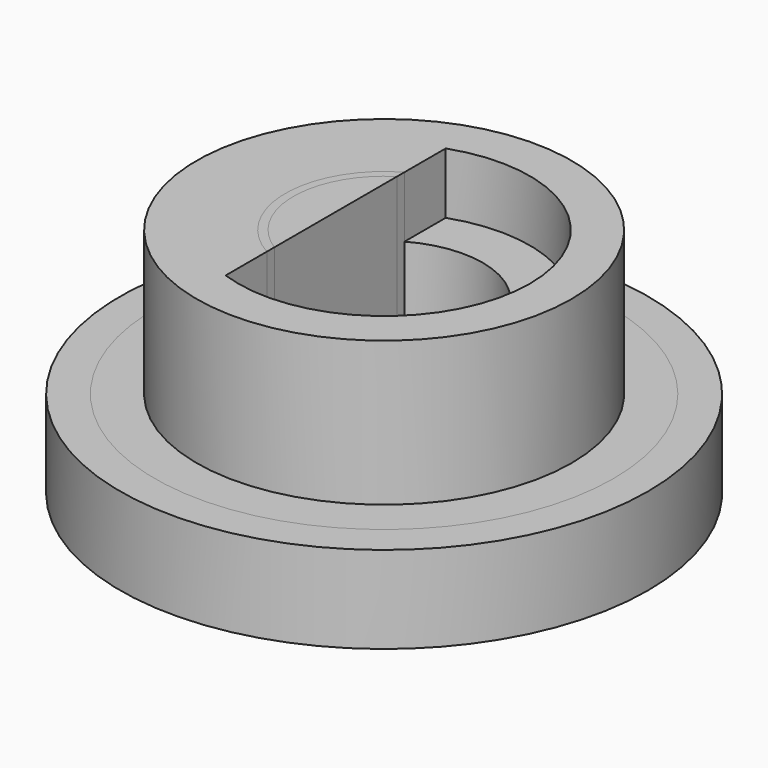
from build123d import *
from build123d import SkipClean  # not in build123d's __all__

# Parameters (mm, degrees)
F1_DEPTH      = 3
F1_DEPTH_BACK = 1
F0_R          = 6.75
F2_DEPTH      = 5.2
F2_DEPTH_BACK = 1
F0_R_2        = 8.26
F3_DEPTH      = 1
F0_R_3        = 9.505
F4_DEPTH      = 3.14
F5_DEPTH      = 5.2
F6_DEPTH      = 5.2
F6_DEPTH_BACK = 1


with BuildPart() as f1:
    # F0 (on Top) → F1 (new body, two sides)
    with BuildSketch(Plane.XY) as f1_sk:
        with BuildLine():
            ThreePointArc((-1.745, 3.0972568508), (1.7936763922, 3.0693240298), (3.555, 0))
            ThreePointArc((3.555, 0), (1.7936763922, -3.0693240298), (-1.745, -3.0972568508))
            Line((-1.745, -3.0972568508), (-1.745, -4.9515123952))
            ThreePointArc((-1.745, -4.9515123952), (3.0332532041, -4.2850758453), (5.25, 0))
            ThreePointArc((5.25, 0), (3.0332532041, 4.2850758453), (-1.745, 4.9515123952))
            Line((-1.745, 4.9515123952), (-1.745, 3.0972568508))
        make_face()
    extrude(amount=F1_DEPTH)
    extrude(f1_sk.sketch, amount=-F1_DEPTH_BACK)

    # F0 (on Top) → F2 (join, two sides)
    with BuildSketch(Plane.XY) as f2_sk:
        Circle(F0_R)
        with BuildLine():
            ThreePointArc((-1.745, -4.9515123952), (-5.25, 0), (-1.745, 4.9515123952))
            ThreePointArc((-1.745, 4.9515123952), (3.0332532041, 4.2850758453), (5.25, 0))
            ThreePointArc((5.25, 0), (3.0332532041, -4.2850758453), (-1.745, -4.9515123952))
        make_face(mode=Mode.SUBTRACT)
        with BuildLine():
            ThreePointArc((-1.745, -3.0972568508), (-3.555, 0), (-1.745, 3.0972568508))
            Line((-1.745, 3.0972568508), (-1.745, 4.9515123952))
            ThreePointArc((-1.745, 4.9515123952), (-5.25, 0), (-1.745, -4.9515123952))
            Line((-1.745, -4.9515123952), (-1.745, -3.0972568508))
        make_face()
    with SkipClean():  # cleaning this boolean's faces spoils the solid; the shape is the same uncleaned
        extrude(amount=F2_DEPTH)
        extrude(f2_sk.sketch, amount=-F2_DEPTH_BACK)


with BuildPart() as f3:
    # F0 (on Top) → F3 (new body)
    with BuildSketch(Plane.XY):
        Circle(F0_R_2)
        Circle(F0_R, mode=Mode.SUBTRACT)
    extrude(amount=-F3_DEPTH)


with BuildPart() as f3b:
    # F0 (on Top) → F3, piece 2 (new body)
    with BuildSketch(Plane.XY):
        with BuildLine():
            Line((-1.745, 0), (2.48, 0))
            ThreePointArc((2.48, 0), (0.9546727188, 2.288886192), (-1.745, 1.7622074225))
            Line((-1.745, 1.7622074225), (-1.745, 0))
        make_face()
        with BuildLine():
            Line((3.265, 0), (3.555, 0))
            ThreePointArc((3.555, 0), (1.7936763922, 3.0693240298), (-1.745, 3.0972568508))
            Line((-1.745, 3.0972568508), (-1.745, 2.7595651831))
            ThreePointArc((-1.745, 2.7595651831), (1.5752460125, 2.8598645073), (3.265, 0))
        make_face()
        with BuildLine():
            ThreePointArc((-1.745, -1.7622074225), (0.9546727188, -2.288886192), (2.48, 0))
            Line((2.48, 0), (-1.745, 0))
            Line((-1.745, 0), (-1.745, -1.7622074225))
        make_face()
        with BuildLine():
            ThreePointArc((-1.745, -2.7595651831), (1.5752460125, -2.8598645073), (3.265, 0))
            Line((3.265, 0), (2.48, 0))
            ThreePointArc((2.48, 0), (0.9546727188, -2.288886192), (-1.745, -1.7622074225))
            Line((-1.745, -1.7622074225), (-1.745, -2.7595651831))
        make_face()
        with BuildLine():
            Line((-1.745, 0), (-1.745, 1.7622074225))
            ThreePointArc((-1.745, 1.7622074225), (-2.48, 0), (-1.745, -1.7622074225))
            Line((-1.745, -1.7622074225), (-1.745, 0))
        make_face()
        with BuildLine():
            Line((-1.745, 1.7622074225), (-1.745, 2.7595651831))
            ThreePointArc((-1.745, 2.7595651831), (-3.265, 0), (-1.745, -2.7595651831))
            Line((-1.745, -2.7595651831), (-1.745, -1.7622074225))
            ThreePointArc((-1.745, -1.7622074225), (-2.48, 0), (-1.745, 1.7622074225))
        make_face()
        with BuildLine():
            ThreePointArc((-1.745, -3.0972568508), (1.7936763922, -3.0693240298), (3.555, 0))
            Line((3.555, 0), (3.265, 0))
            ThreePointArc((3.265, 0), (1.5752460125, -2.8598645073), (-1.745, -2.7595651831))
            Line((-1.745, -2.7595651831), (-1.745, -3.0972568508))
        make_face()
        with BuildLine():
            Line((2.48, 0), (3.265, 0))
            ThreePointArc((3.265, 0), (1.5752460125, 2.8598645073), (-1.745, 2.7595651831))
            Line((-1.745, 2.7595651831), (-1.745, 1.7622074225))
            ThreePointArc((-1.745, 1.7622074225), (0.9546727188, 2.288886192), (2.48, 0))
        make_face()
        with BuildLine():
            ThreePointArc((-1.745, -3.0972568508), (-3.555, 0), (-1.745, 3.0972568508))
            Line((-1.745, 3.0972568508), (-1.745, 4.9515123952))
            ThreePointArc((-1.745, 4.9515123952), (-5.25, 0), (-1.745, -4.9515123952))
            Line((-1.745, -4.9515123952), (-1.745, -3.0972568508))
        make_face()
        with BuildLine():
            Line((-1.745, 2.7595651831), (-1.745, 3.0972568508))
            ThreePointArc((-1.745, 3.0972568508), (-3.555, 0), (-1.745, -3.0972568508))
            Line((-1.745, -3.0972568508), (-1.745, -2.7595651831))
            ThreePointArc((-1.745, -2.7595651831), (-3.265, 0), (-1.745, 2.7595651831))
        make_face()
    extrude(amount=-F3_DEPTH)


with BuildPart() as f4:
    # F0 (on Top) → F4 (new body)
    with BuildSketch(Plane.XY):
        Circle(F0_R_3)
        Circle(F0_R_2, mode=Mode.SUBTRACT)
    extrude(amount=-F4_DEPTH)


with BuildPart() as f5:
    # F0 (on Top) → F5 (new body)
    with BuildSketch(Plane.XY):
        with BuildLine():
            Line((-1.745, 2.7595651831), (-1.745, 3.0972568508))
            ThreePointArc((-1.745, 3.0972568508), (-3.555, 0), (-1.745, -3.0972568508))
            Line((-1.745, -3.0972568508), (-1.745, -2.7595651831))
            ThreePointArc((-1.745, -2.7595651831), (-3.265, 0), (-1.745, 2.7595651831))
        make_face()
    extrude(amount=F5_DEPTH)


with BuildPart() as f6:
    # F0 (on Top) → F6 (new body, two sides)
    with BuildSketch(Plane.XY) as f6_sk:
        with BuildLine():
            Line((-1.745, 1.7622074225), (-1.745, 2.7595651831))
            ThreePointArc((-1.745, 2.7595651831), (-3.265, 0), (-1.745, -2.7595651831))
            Line((-1.745, -2.7595651831), (-1.745, -1.7622074225))
            ThreePointArc((-1.745, -1.7622074225), (-2.48, 0), (-1.745, 1.7622074225))
        make_face()
        with BuildLine():
            Line((-1.745, 0), (-1.745, 1.7622074225))
            ThreePointArc((-1.745, 1.7622074225), (-2.48, 0), (-1.745, -1.7622074225))
            Line((-1.745, -1.7622074225), (-1.745, 0))
        make_face()
    extrude(amount=F6_DEPTH)
    extrude(f6_sk.sketch, amount=-F6_DEPTH_BACK)


solid = Compound([f1.part, f3.part, f3b.part, f4.part, f5.part, f6.part])
